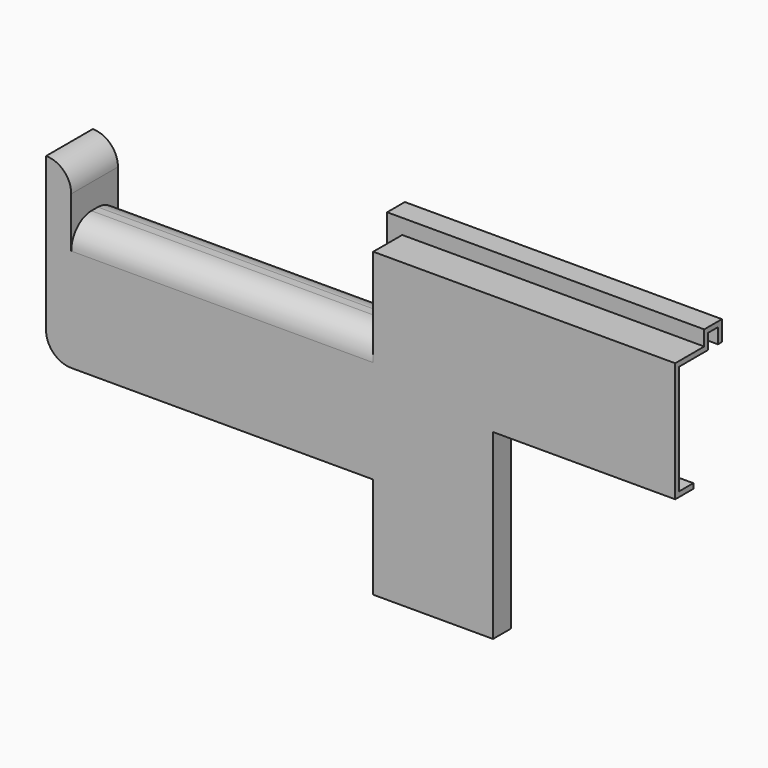
from build123d import *

# Parameters (mm, degrees)
F0_W         = 23.8
F0_H         = 23.8
F0_W_2       = 36.2
F0_H_2       = 36.2
F1_DEPTH     = 1
F2_W         = 59
F2_H         = 1
F2_W_2       = 1
F2_H_2       = 59
F3_DEPTH     = 7.2
F4_W         = 36.2
F4_H         = 1
F5_DEPTH     = 3.5
F6_W         = 60
F6_H         = 1
F7_DEPTH     = 3
F8_W         = 60
F8_H         = 1
F9_DEPTH     = 3.4
F10_W        = 60
F10_H        = 1
F11_DEPTH    = 3
F12_W        = 1
F12_H        = 60
F13_DEPTH    = 3
F14_W        = 1
F14_H        = 60
F15_DEPTH    = 3.4
F16_W        = 1
F16_H        = 60
F17_DEPTH    = 3
F18_DEPTH    = 3
F19_DEPTH    = 2
F20_W        = 7.2
F20_H        = 25.4523856565
F21_DEPTH    = 65
F22_W        = 4.4
F22_H        = 25.4523856565
F23_DEPTH    = 62
F24_W        = 5
F24_H        = 11.6
F25_DEPTH    = 10
F26_R        = 4.99999
F27_T1_DEPTH = 60
F27_T3_DEPTH = 57
F27_T8_DEPTH = 69.5
F28_R        = 5


# Not quite as in the source:
# - a fillet or chamfer that OpenCascade refuses, or shapes differently, is made with other operations: its cross-section is extruded or revolved along the edge and cut away or added
# - a fillet or chamfer is up to 0.001 mm smaller than in the source, because OpenCascade refuses the exact size


with BuildPart() as f1:
    # F0 (on Front) → F1 (new body)
    with BuildSketch(Plane.XZ):
        with Locations((-18.1, 18.1)):
            Rectangle(F0_W, F0_H)
        with Locations((11.9, 18.1)):
            Rectangle(F0_W_2, F0_H)
        with Locations((-18.1, -11.9)):
            Rectangle(F0_W, F0_H_2)
    extrude(amount=F1_DEPTH)

    # F2 (on face) → F3 (join)
    with BuildSketch(Plane(origin=(0, 0, 0), x_dir=(-1, 0, 0), z_dir=(0, 1, 0))):
        with Locations((-0.5, 29.5)):
            Rectangle(F2_W, F2_H)
        with Locations((29.5, 29.5)):
            Rectangle(F2_W_2, F2_H)
        with Locations((29.5, -0.5)):
            Rectangle(F2_W_2, F2_H_2)
    extrude(amount=F3_DEPTH)

    # F4 (on face) → F5 (join)
    with BuildSketch(Plane(origin=(0, 0, 0), x_dir=(-1, 0, 0), z_dir=(0, 1, 0))):
        with Locations((-11.9, 6.7)):
            Rectangle(F4_W, F4_H)
        Polygon((6.2, 7.2), (6.2, 6.2), (6.2, -30), (7.2, -30), (7.2, 7.2), align=None)
    extrude(amount=F5_DEPTH)

    # F6 (on face) → F7 (join)
    with BuildSketch(Plane.XY.offset(30)):
        with Locations((0, 6.7)):
            Rectangle(F6_W, F6_H)
    extrude(amount=F7_DEPTH)

    # F8 (on face) → F9 (join)
    with BuildSketch(Plane(origin=(0, 7.2, 0), x_dir=(-1, 0, 0), z_dir=(0, 1, 0))):
        with Locations((0, 32.5)):
            Rectangle(F8_W, F8_H)
    extrude(amount=F9_DEPTH)

    # F10 (on face) → F11 (join)
    with BuildSketch(Plane(origin=(0, 0, 32), x_dir=(1, 0, 0), z_dir=(0, 0, -1))):
        with Locations((0, -10.1)):
            Rectangle(F10_W, F10_H)
    extrude(amount=F11_DEPTH)

    # F12 (on face) → F13 (join)
    with BuildSketch(Plane(origin=(-30, 0, 0), x_dir=(0, -1, 0), z_dir=(-1, 0, 0))):
        with Locations((-6.7, 0)):
            Rectangle(F12_W, F12_H)
    extrude(amount=F13_DEPTH)

    # F14 (on face) → F15 (join)
    with BuildSketch(Plane(origin=(0, 7.2, 0), x_dir=(-1, 0, 0), z_dir=(0, 1, 0))):
        with Locations((32.5, 0)):
            Rectangle(F14_W, F14_H)
    extrude(amount=F15_DEPTH)

    # F16 (on face) → F17 (join)
    with BuildSketch(Plane.YZ.offset(-32)):
        with Locations((10.1, 0)):
            Rectangle(F16_W, F16_H)
    extrude(amount=F17_DEPTH)

    # F18 (add): a face of the model
    f18_faces = [f1.faces().sort_by_distance(p)[0] for p in [
        (-30, 6.2532541078, 31.5),
    ]]
    extrude(f18_faces, amount=F18_DEPTH)

    # F19 (add): a face of the model
    f19_faces = [f1.faces().sort_by_distance(p)[0] for p in [
        (-32.5, 8.4, 30),
    ]]
    extrude(f19_faces, amount=F19_DEPTH)

    # F20 (on face) → F21 (join)
    with BuildSketch(Plane(origin=(-30, 0, 0), x_dir=(0, -1, 0), z_dir=(-1, 0, 0))):
        with Locations((-2.6, 2.8769155033)):
            Rectangle(F20_W, F20_H)
    extrude(amount=F21_DEPTH)

    # F22 (on face) → F23 (join)
    with BuildSketch(Plane(origin=(-33, 0, 0), x_dir=(0, -1, 0), z_dir=(-1, 0, 0))):
        with Locations((-8.4, 2.8769155033)):
            Rectangle(F22_W, F22_H)
    extrude(amount=F23_DEPTH)

    # F24 (on face) → F25 (join)
    with BuildSketch(Plane.XY.offset(15.6031083316)):
        with Locations((-92.5, 4.8)):
            Rectangle(F24_W, F24_H)
    extrude(amount=F25_DEPTH)

    # F26 (radius 5 in the source; OpenCascade refuses exactly that, so slightly less here)
    f26_edges = [f1.edges().sort_by_distance(p)[0] for p in [
        (-90, 4.8, 25.603108),
    ]]
    fillet(f26_edges, radius=F26_R)

    # F27: fillet of radius 5 on 2 edges, made by hand

    # F27_s2 → F27_t1 (cut)
    with BuildSketch(Plane.YZ.offset(-90)):
        with BuildLine():
            ThreePointArc((-1, 10.6031083316), (0.4644660941, 14.1386422375), (4, 15.6031083316))
            Line((4, 15.6031083316), (-1, 15.6031083316))
            Line((-1, 15.6031083316), (-1, 10.6031083316))
        make_face()
    extrude(amount=F27_T1_DEPTH, mode=Mode.SUBTRACT)

    # F27_s4 → F27_t3 (cut)
    with BuildSketch(Plane.YZ.offset(-90)):
        with BuildLine():
            ThreePointArc((5.6, 15.6031083316), (9.1355339059, 14.1386422375), (10.6, 10.6031083316))
            Line((10.6, 10.6031083316), (10.6, 15.6031083316))
            Line((10.6, 15.6031083316), (5.6, 15.6031083316))
        make_face()
    extrude(amount=F27_T3_DEPTH, mode=Mode.SUBTRACT)


with BuildPart() as f27_tool6:
    # F27_s7 → F27_t8 (new body)
    with BuildSketch(Plane.YZ.offset(-20.5)):
        with BuildLine():
            ThreePointArc((5.6, 15.6031083316), (9.1355339059, 14.1386422375), (10.6, 10.6031083316))
            Line((10.6, 10.6031083316), (10.6, 15.6031083316))
            Line((10.6, 15.6031083316), (5.6, 15.6031083316))
        make_face()
    extrude(amount=-F27_T8_DEPTH)

    split(bisect_by=Plane.YZ.offset(-30), keep=Keep.BOTTOM)

    split(bisect_by=Plane.XZ.offset(-6.2), keep=Keep.TOP)


with BuildPart() as f1_1:
    add(f1.part)

    # F27_t5: cut F27_tool6
    add(f27_tool6.part, mode=Mode.SUBTRACT)

    # F28
    f28_edges = [f1_1.edges().sort_by_distance(p)[0] for p in [
        (-95, 4.8, -9.849277),
    ]]
    fillet(f28_edges, radius=F28_R)


solid = f1_1.part
